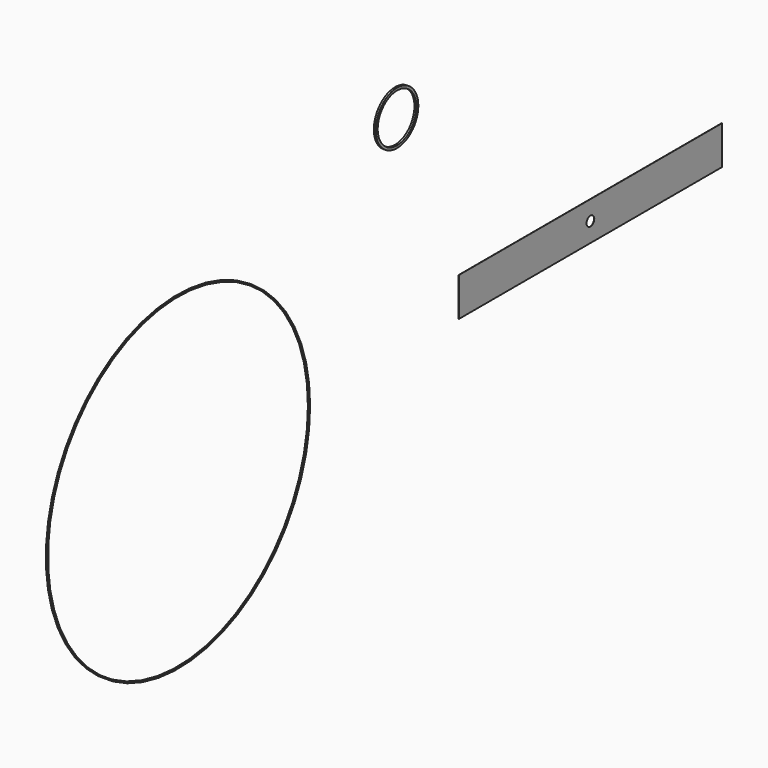
from build123d import *

# Parameters (mm, degrees)
F0_W     = 431.8
F0_H     = 50.8
F0_R     = 6.35
F1_DEPTH = 0.254
F2_R     = 215.9
F2_R_2   = 214.3125
F3_DEPTH = 1.5875
F4_R     = 34.925
F4_R_2   = 31.75
F5_DEPTH = 2.54


# Not quite as in the source:
# - a feature names something its author has since deleted; it is built from what else it names


with BuildPart() as f1:
    # F0 (on Right) → F1 (new body)
    with BuildSketch(Plane.YZ):
        with Locations((215.9, 25.4)):
            Rectangle(F0_W, F0_H)
        with Locations((215.9, 25.4)):
            Circle(F0_R, mode=Mode.SUBTRACT)
    extrude(amount=F1_DEPTH)


with BuildPart() as f3:
    # F2 (on Right) → F3 (new body)
    with BuildSketch(Plane.YZ):
        with Locations((-461.7941379547, 0)):
            Circle(F2_R)
        with Locations((-461.7941379547, 0)):
            Circle(F2_R_2, mode=Mode.SUBTRACT)
    extrude(amount=F3_DEPTH)


with BuildPart() as f5:
    # F4 (on Right) → F5 (new body)
    with BuildSketch(Plane.YZ):
        with Locations((-104.3467223644, 275.5787670612)):
            Circle(F4_R)
        with Locations((-104.3467223644, 275.5787670612)):
            Circle(F4_R_2, mode=Mode.SUBTRACT)
    extrude(amount=F5_DEPTH)


solid = Compound([f1.part, f3.part, f5.part])
